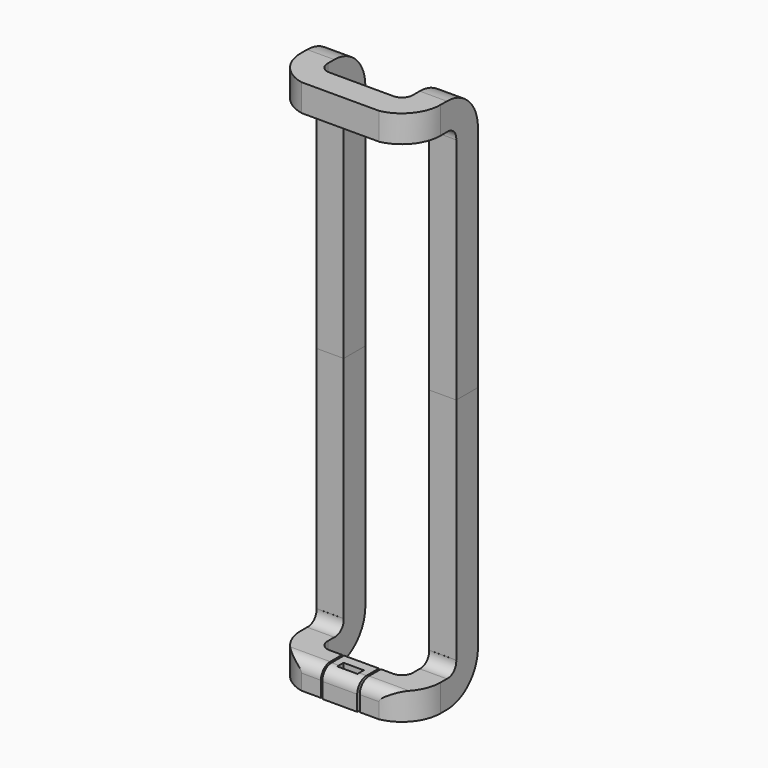
from build123d import *

# Parameters (mm, degrees)
F3_DEPTH      = 69
F4_W          = 9.8017244339
F4_H          = 7
F5_DEPTH      = 81.7
F7_W          = 9
F7_H          = 7
F7_W_2        = 5.2275949775
F7_H_2        = 1.981525898
F8_DEPTH      = 7
F9_T1_DEPTH   = 19.9814636312
F9_2_T1_DEPTH = 19.9814636312
F9_3_T1_DEPTH = 24
F10_DEPTH     = 11.5


# Not quite as in the source:
# - a fillet or chamfer that OpenCascade refuses, or shapes differently, is made with other operations: its cross-section is extruded or revolved along the edge and cut away or added


with BuildPart() as f3:
    # F2 (on Top) → F3 (new body)
    with BuildSketch(Plane.XY):
        with BuildLine():
            Line((-126.34694054, 507.5408363342), (-126.34694054, 500.5408363342))
            Line((-126.34694054, 500.5408363342), (-126.34694054, 495.5408363342))
            ThreePointArc((-126.34694054, 495.5408363342), (-123.4180083519, 488.4697685224), (-116.34694054, 485.5408363342))
            Line((-116.34694054, 485.5408363342), (-113.34694054, 485.5408363342))
            Line((-113.34694054, 485.5408363342), (-113.34694054, 492.5408363342))
            Line((-113.34694054, 492.5408363342), (-116.34694054, 492.5408363342))
            ThreePointArc((-116.34694054, 492.5408363342), (-118.5323459538, 493.3554309204), (-119.34694054, 495.5408363342))
            Line((-119.34694054, 495.5408363342), (-119.34694054, 500.5408363342))
            Line((-119.34694054, 500.5408363342), (-119.34694054, 507.5408363342))
            Line((-119.34694054, 507.5408363342), (-126.34694054, 507.5408363342))
        make_face()
    extrude(amount=F3_DEPTH)


with BuildPart() as f3b:
    # F2 (on Top) → F3, piece 2 (new body)
    with BuildSketch(Plane.XY):
        with BuildLine():
            Line((-103.34694054, 492.5408363342), (-103.34694054, 485.5408363342))
            Line((-103.34694054, 485.5408363342), (-100.34694054, 485.5408363342))
            ThreePointArc((-100.34694054, 485.5408363342), (-93.2758727282, 488.4697685224), (-90.34694054, 495.5408363342))
            Line((-90.34694054, 495.5408363342), (-90.34694054, 500.5408363342))
            Line((-90.34694054, 500.5408363342), (-90.34694054, 507.5408363342))
            Line((-90.34694054, 507.5408363342), (-97.34694054, 507.5408363342))
            Line((-97.34694054, 507.5408363342), (-97.34694054, 500.5408363342))
            Line((-97.34694054, 500.5408363342), (-97.34694054, 495.5408363342))
            ThreePointArc((-97.34694054, 495.5408363342), (-98.1615351262, 493.3554309204), (-100.34694054, 492.5408363342))
            Line((-100.34694054, 492.5408363342), (-103.34694054, 492.5408363342))
        make_face()
    extrude(amount=F3_DEPTH)


with BuildPart() as f5_tool:
    # F4 (on face) → F5 (new body)
    with BuildSketch(Plane(origin=(-126.34694054, 0, 0), x_dir=(0, -1, 0), z_dir=(-1, 0, 0))):
        Polygon((-500.5727462455, 69), (-507.5408363342, 69), (-507.5408363342, 16.4578538388), (-507.5408363342, 10), (-500.5727462455, 10), align=None)
        with Locations((-490.6399741173, 3.5)):
            Rectangle(F4_W, F4_H)
        with BuildLine():
            Line((-500.5599826709, 10), (-500.5727462455, 10))
            Line((-500.5727462455, 10), (-507.5408363342, 10))
            ThreePointArc((-507.5408363342, 10), (-504.6119041461, 2.9289321881), (-497.5408363342, 0))
            Line((-497.5408363342, 0), (-495.5408363342, 0))
            Line((-495.5408363342, 0), (-495.5408363342, 7))
            Line((-495.5408363342, 7), (-497.5408363342, 7))
            ThreePointArc((-497.5408363342, 7), (-499.7591459044, 7.7867403629), (-500.5599826709, 10))
        make_face()
    extrude(amount=-F5_DEPTH)


with BuildPart() as f3_1:
    add(f3.part)

    # F5: intersect by f5_tool
    add(f5_tool.part, mode=Mode.INTERSECT)


with BuildPart() as f3b_1:
    add(f3b.part)

    # F5: intersect by f5_tool
    add(f5_tool.part, mode=Mode.INTERSECT)


with BuildPart() as f6_1:
    # F6: instance of F3
    add(f3_1.part.mirror(Plane(origin=(-93.84694054, 504.0567912899, 69), x_dir=(1, 0, 0), z_dir=(0, 0, 1))))



with BuildPart() as f6_2:
    # F6: instance of F3b
    add(f3b_1.part.mirror(Plane(origin=(-93.84694054, 504.0567912899, 69), x_dir=(1, 0, 0), z_dir=(0, 0, 1))))


with BuildPart() as f8:
    # F7 (on Top) → F8 (new body)
    with BuildSketch(Plane.XY):
        with Locations((-108.34694054, 489.0408363342)):
            Rectangle(F7_W, F7_H)
        with Locations((-108.34694054, 489.0408363342)):
            Rectangle(F7_W_2, F7_H_2, mode=Mode.SUBTRACT)
    extrude(amount=F8_DEPTH)

    # F9#3: fillet of radius 3 on 1 edges, made by hand

    # F9_3_s2 → F9_3_t1 (cut)
    with BuildSketch(Plane.YZ.offset(-120.34694054)):
        with BuildLine():
            ThreePointArc((485.5408363342, 4), (486.4195159907, 6.1213203436), (488.5408363342, 7))
            Line((488.5408363342, 7), (485.5408363342, 7))
            Line((485.5408363342, 7), (485.5408363342, 4))
        make_face()
    extrude(amount=F9_3_T1_DEPTH, mode=Mode.SUBTRACT)


with BuildPart() as f3_2:
    add(f3_1.part)

    # F9: fillet of radius 3 on 1 edges, made by hand

    # F9_s2 → F9_t1 (cut)
    with BuildSketch(Plane.YZ.offset(-125.8284041713)):
        with BuildLine():
            ThreePointArc((488.7391119003, 7), (486.6177915568, 6.1213203436), (485.7391119003, 4))
            Line((485.7391119003, 4), (485.7391119003, 7))
            Line((485.7391119003, 7), (488.7391119003, 7))
        make_face()
    extrude(amount=F9_T1_DEPTH, mode=Mode.SUBTRACT)


with BuildPart() as f3b_2:
    add(f3b_1.part)

    # F9#2: fillet of radius 3 on 1 edges, made by hand

    # F9_2_s2 → F9_2_t1 (cut)
    with BuildSketch(Plane.YZ.offset(-110.84694054)):
        with BuildLine():
            ThreePointArc((488.7391119003, 7), (486.6177915568, 6.1213203436), (485.7391119003, 4))
            Line((485.7391119003, 4), (485.7391119003, 7))
            Line((485.7391119003, 7), (488.7391119003, 7))
        make_face()
    extrude(amount=F9_2_T1_DEPTH, mode=Mode.SUBTRACT)


with BuildPart() as f6_1_1:
    add(f6_1.part)
    # F10 (add): a face of the model
    f10_faces = [f6_2.part.faces().sort_by_distance(p)[0] for p in [
        (-103.34694054, 489.1399741173, 134.5),
    ]]

    add(f6_2.part)  # F10 merges F6_2
    extrude(f10_faces, amount=F10_DEPTH)


solid = Compound([f8.part, f3_2.part, f3b_2.part, f6_1_1.part])
